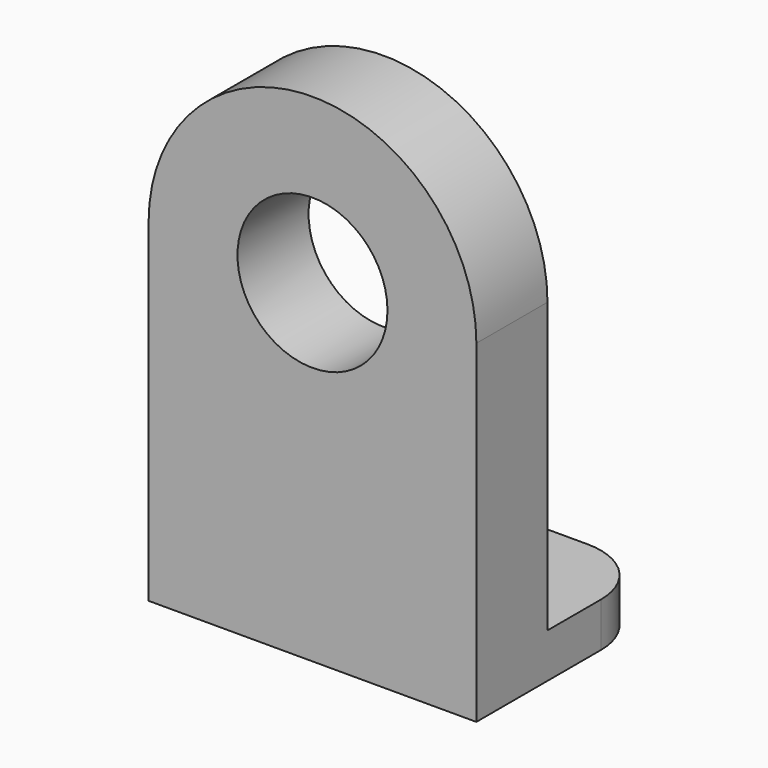
from build123d import *

# Parameters (mm, degrees)
F0_R     = 3.375
F1_DEPTH = 4
F2_W     = 14.75
F2_H     = 6
F2_H_2   = 4
F3_DEPTH = 2
F4_R     = 3
F5_D     = 3


# Not quite as in the source:
# - a feature names something its author has since deleted; it is built from what else it names


with BuildPart() as f1:
    # F0 (on Front) → F1 (new body)
    with BuildSketch(Plane.XZ):
        with BuildLine():
            Line((7.375, -15), (7.375, 0))
            ThreePointArc((7.375, 0), (0, -7.375), (-7.375, 0))
            Line((-7.375, 0), (-7.375, -15))
            Line((-7.375, -15), (7.375, -15))
        make_face()
        with BuildLine():
            ThreePointArc((-7.375, 0), (0, -7.375), (7.375, 0))
            ThreePointArc((7.375, 0), (0, 7.375), (-7.375, 0))
        make_face()
        Circle(F0_R, mode=Mode.SUBTRACT)
    extrude(amount=F1_DEPTH)

    # F2 (on face) → F3 (join)
    with BuildSketch(Plane(origin=(0, 0, -15), x_dir=(1, 0, 0), z_dir=(0, 0, -1))):
        with Locations((0, -3)):
            Rectangle(F2_W, F2_H)
        with Locations((0, 2)):
            Rectangle(F2_W, F2_H_2)
    extrude(amount=-F3_DEPTH)

    # F4
    f4_edges = [f1.edges().sort_by_distance(p)[0] for p in [
        (-7.375, 6, -14),
        (7.375, 6, -14),
    ]]
    fillet(f4_edges, radius=F4_R)

    # F5 (through all)
    with Locations(Plane(origin=(0, 0, -15), x_dir=(1, 0, 0), z_dir=(0, 0, -1))):
        with Locations((0, -3)):
            Hole(F5_D / 2)


solid = f1.part
